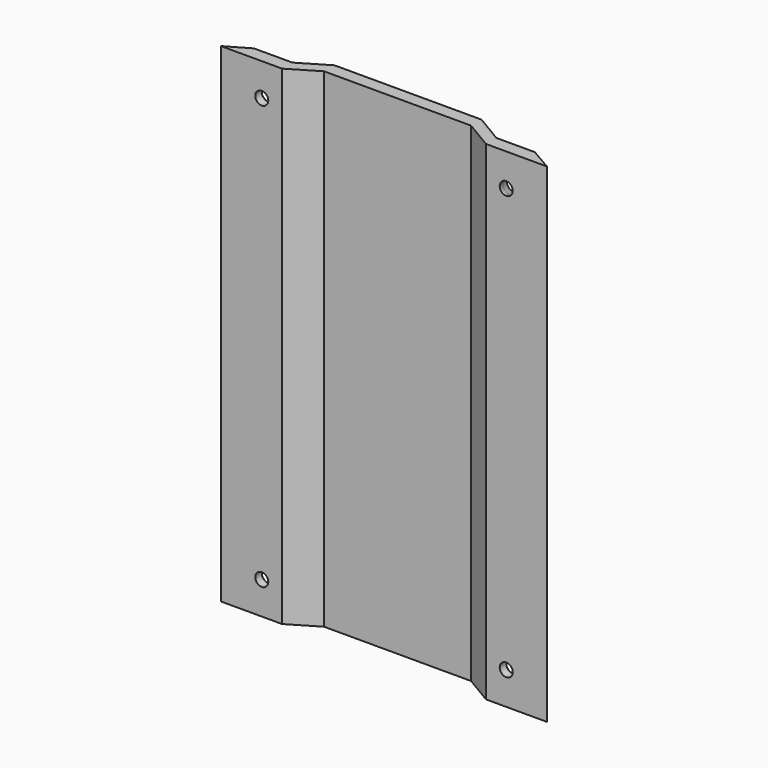
from build123d import *

# Parameters (mm, degrees)
F0_W     = 22.5599961265
F0_H     = 4
F1_DEPTH = 150
F2_R     = 2
F3_DEPTH = 9.20100235
F4_SIZE  = 1


# Not quite as in the source:
# - a fillet or chamfer that OpenCascade refuses, or shapes differently, is made with other operations: its cross-section is extruded or revolved along the edge and cut away or added


with BuildPart() as f1:
    # F0 (on Top) → F1 (new body)
    with BuildSketch(Plane.XY):
        Polygon((0, -4), (0, 0), (-8.7200025445, -5.20000235), (-20.5118006432, -5.20000235), (-27.4400038735, -9.20000235), (-8.7200025445, -9.20000235), align=None)
        with Locations((11.2799980633, -2)):
            Rectangle(F0_W, F0_H)
        with Locations((33.8399941898, -2)):
            Rectangle(F0_W, F0_H)
        Polygon((53.8399947975, -5.20000235), (45.119992253, 0), (45.119992253, -4), (53.8399947975, -9.20000235), (72.5599961265, -9.20000235), (65.6317928962, -5.20000235), align=None)
    extrude(amount=F1_DEPTH)

    # F2 (on face) → F3 (cut, through all)
    with BuildSketch(Plane.XZ.offset(9.20000235)):
        with Locations((-14.9400038735, 140)):
            Circle(F2_R)
        with Locations((60.0599961265, 140)):
            Circle(F2_R)
        with Locations((-14.9400038735, 10)):
            Circle(F2_R)
        with Locations((60.0599961265, 10)):
            Circle(F2_R)
    extrude(amount=-F3_DEPTH, mode=Mode.SUBTRACT)

    # F4
    f4_edges = [f1.edges().sort_by_distance(p)[0] for p in [
        (58.059996, -5.200002, 140),
    ]]
    chamfer(f4_edges, length=F4_SIZE)

    # F5: chamfer of 2 on 1 edges, made by hand

    # F5_s1 → F5_t2 (revolve, cut)
    with BuildSketch(Plane.XY.offset(140)):
        Polygon((63.4742096889, -4.7857887876), (62.0599961265, -8.20000235), (62.0599961265, -6.20000235), align=None)
    revolve(axis=Axis((60.0599961265, -6.20000235, 140), (0, -1, 0)), mode=Mode.SUBTRACT)

    # F6: chamfer of 1.5 on 4 edges, made by hand

    # F6_s1 → F6_t2 (revolve, cut)
    with BuildSketch(Plane.XY.offset(10)):
        Polygon((63.5599961265, -5.20000235), (62.0599961265, -6.70000235), (62.0599961265, -5.20000235), align=None)
    revolve(axis=Axis((60.0599961265, -5.20000235, 10), (0, -1, 0)), mode=Mode.SUBTRACT)

    # F6_s3 → F6_t4 (revolve, cut)
    with BuildSketch(Plane.XY.offset(10)):
        Polygon((-11.4400038735, -5.20000235), (-12.9400038735, -6.70000235), (-12.9400038735, -5.20000235), align=None)
    revolve(axis=Axis((-14.9400038735, -5.20000235, 10), (0, -1, 0)), mode=Mode.SUBTRACT)

    # F6_s5 → F6_t6 (revolve, cut)
    with BuildSketch(Plane.XY.offset(140)):
        Polygon((-11.4400038735, -5.20000235), (-12.9400038735, -6.70000235), (-12.9400038735, -5.20000235), align=None)
    revolve(axis=Axis((-14.9400038735, -5.20000235, 140), (0, -1, 0)), mode=Mode.SUBTRACT)

    # F6_s7 → F6_t8 (revolve, cut)
    with BuildSketch(Plane.XY.offset(140)):
        Polygon((62.1741768278, -7.9243457525), (62.0599961265, -8.498370901), (62.0599961265, -8.20000235), align=None)
    revolve(axis=Axis((60.0599961265, -8.20000235, 140), (0, -1, 0)), mode=Mode.SUBTRACT)


solid = f1.part
